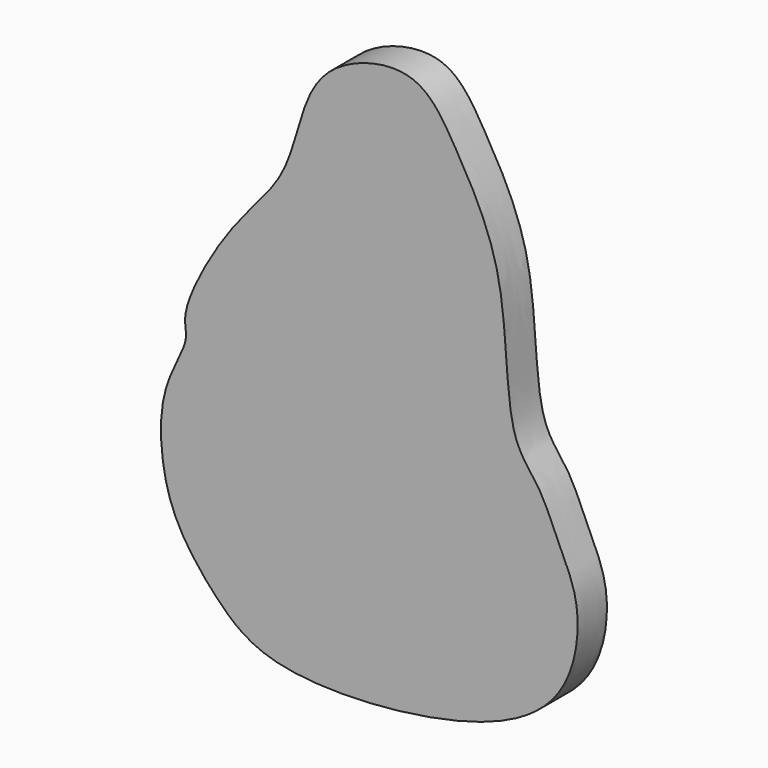
from build123d import *

# Parameters (mm, degrees)
F1_DEPTH = 6.35


# Not quite as in the source:
# - a feature names something its author has since deleted; it is built from what else it names


with BuildPart() as f1:
    # F0 (on Front) → F1 (new body)
    with BuildSketch(Plane.XZ):
        with BuildLine():
            add(Edge.make_bspline(
                [(-27.6293512434, 0), (-27.1172896263, 3.5376254392), (-20.2092513225, 16.3072133999), (-10.8392504403, 25.1467404672), (-8.0747318133, 34.8434785474), (-4.5300661972, 46.7069107339), (12.6075059031, 51.7105715763), (19.7257277224, 39.9676667182), (28.7779451774, 24.0962644882), (27.6740258612, -0.421871611), (34.0813959728, -6.1160111709), (37.0282916957, -14.1238412328), (41.5566608206, -22.2388548115), (39.2860211775, -38.9719075539), (20.1943249395, -48.8609336235), (-12.4163877173, -50.5797798703), (-21.8081226127, -42.4979054548), (-28.0357268673, -34.9114485477), (-31.7514062662, -26.6618791131), (-32.58384075, -12.6907975978), (-26.6389070636, -4.129267785), (-27.8777750886, -1.716259304), (-27.6293512434, 0)],
                knots=[0, 0, 0, 0, 0.0578515626, 0.1092828013, 0.1525307013, 0.2003889319, 0.2532875978, 0.3009135883, 0.3619956922, 0.4293468962, 0.468276435, 0.5077773412, 0.5501787861, 0.6032246174, 0.6667396033, 0.7454404961, 0.7928604617, 0.8353038116, 0.8773265245, 0.9292953295, 0.9719336362, 1, 1, 1, 1], degree=3))
        make_face()
    extrude(amount=F1_DEPTH)


solid = f1.part
